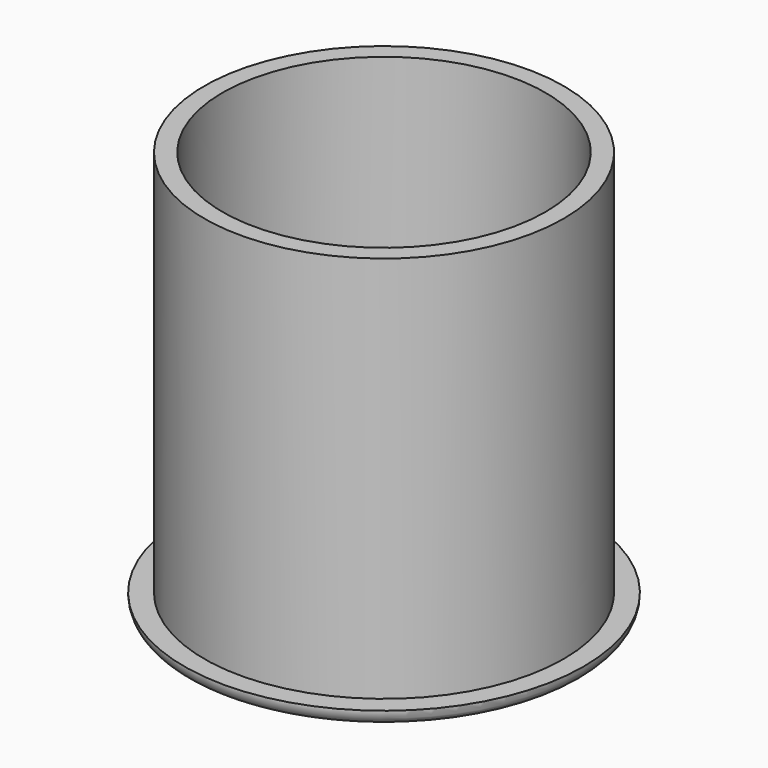
from build123d import *

# Parameters (mm, degrees)
F0_R     = 22.25
F0_R_2   = 20
F1_DEPTH = 50
F0_R_3   = 24.75
F2_DEPTH = 2
F3_R     = 1.99999


# Not quite as in the source:
# - a fillet or chamfer is up to 0.001 mm smaller than in the source, because OpenCascade refuses the exact size


with BuildPart() as f1:
    # F0 (on Top) → F1 (new body)
    with BuildSketch(Plane.XY):
        Circle(F0_R)
        Circle(F0_R_2, mode=Mode.SUBTRACT)
    extrude(amount=F1_DEPTH)

    # F0 (on Top) → F2 (join)
    with BuildSketch(Plane.XY):
        Circle(F0_R_3)
        Circle(F0_R, mode=Mode.SUBTRACT)
    extrude(amount=F2_DEPTH)

    # F3 (radius 2 in the source; OpenCascade refuses exactly that, so slightly less here)
    f3_edges = [f1.edges().sort_by_distance(p)[0] for p in [
        (-24.75, 0, 0),
    ]]
    fillet(f3_edges, radius=F3_R)


solid = f1.part
